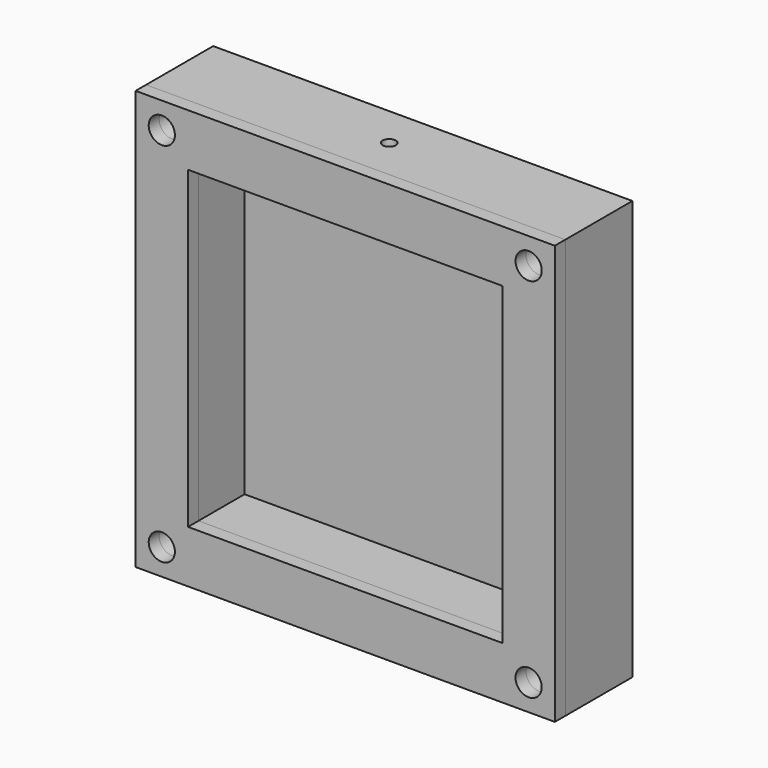
from build123d import *

# Parameters (mm, degrees)
F0_R     = 3.175
F0_W     = 12.7
F0_H     = 12.7
F1_DEPTH = 6.35
F2_DEPTH = 20.32
F3_R     = 1.5875
F4_DEPTH = 25.4
F5_W     = 101.6
F5_H     = 101.6
F5_R     = 3.175
F5_W_2   = 76.2
F5_H_2   = 76.2
F6_DEPTH = 3.175


# Not quite as in the source:
# - a feature names something its author has since deleted; it is built from what else it names


with BuildPart() as f1:
    # F0 (on Front) → F1 (new body)
    with BuildSketch(Plane.XZ):
        Polygon((38.1, 38.1), (38.1, 0), (38.1, -38.1), (-38.1, -38.1), (-38.1, 0), (-38.1, 38.1), (-50.8, 38.1), (-50.8, -50.8), (50.8, -50.8), (50.8, 38.1), align=None)
        with Locations((-44.45, -44.45)):
            Circle(F0_R, mode=Mode.SUBTRACT)
        with Locations((44.45, -44.45)):
            Circle(F0_R, mode=Mode.SUBTRACT)
        Polygon((38.1, -38.1), (38.1, 0), (38.1, 38.1), (0, 38.1), (-38.1, 38.1), (-38.1, 0), (-38.1, -38.1), align=None)
        Polygon((0, 38.1), (38.1, 38.1), (38.1, 50.8), (-38.1, 50.8), (-38.1, 38.1), align=None)
        with Locations((-44.45, 44.45)):
            Rectangle(F0_W, F0_H)
        with Locations((-44.45, 44.45)):
            Circle(F0_R, mode=Mode.SUBTRACT)
        with Locations((44.45, 44.45)):
            Rectangle(F0_W, F0_H)
        with Locations((44.45, 44.45)):
            Circle(F0_R, mode=Mode.SUBTRACT)
    extrude(amount=F1_DEPTH)

    # F0 (on Front) → F2 (join)
    with BuildSketch(Plane.XZ):
        Polygon((38.1, 38.1), (38.1, 0), (38.1, -38.1), (-38.1, -38.1), (-38.1, 0), (-38.1, 38.1), (-50.8, 38.1), (-50.8, -50.8), (50.8, -50.8), (50.8, 38.1), align=None)
        with Locations((-44.45, -44.45)):
            Circle(F0_R, mode=Mode.SUBTRACT)
        with Locations((44.45, -44.45)):
            Circle(F0_R, mode=Mode.SUBTRACT)
        Polygon((0, 38.1), (38.1, 38.1), (38.1, 50.8), (-38.1, 50.8), (-38.1, 38.1), align=None)
        with Locations((44.45, 44.45)):
            Rectangle(F0_W, F0_H)
        with Locations((44.45, 44.45)):
            Circle(F0_R, mode=Mode.SUBTRACT)
        with Locations((-44.45, 44.45)):
            Rectangle(F0_W, F0_H)
        with Locations((-44.45, 44.45)):
            Circle(F0_R, mode=Mode.SUBTRACT)
    extrude(amount=F2_DEPTH)

    # F3 (on face) → F4 (cut)
    with BuildSketch(Plane.XY.offset(50.8)):
        with Locations((0, -10.16)):
            Circle(F3_R)
    extrude(amount=-F4_DEPTH, mode=Mode.SUBTRACT)


with BuildPart() as f6:
    # F5 (on face) → F6 (new body)
    with BuildSketch(Plane.XZ.offset(20.32)):
        Rectangle(F5_W, F5_H)
        with Locations((-44.45, -44.45)):
            Circle(F5_R, mode=Mode.SUBTRACT)
        Rectangle(F5_W_2, F5_H_2, mode=Mode.SUBTRACT)
        with Locations((44.45, -44.45)):
            Circle(F5_R, mode=Mode.SUBTRACT)
        with Locations((-44.45, 44.45)):
            Circle(F5_R, mode=Mode.SUBTRACT)
        with Locations((44.45, 44.45)):
            Circle(F5_R, mode=Mode.SUBTRACT)
    extrude(amount=F6_DEPTH)


solid = Compound([f1.part, f6.part])
